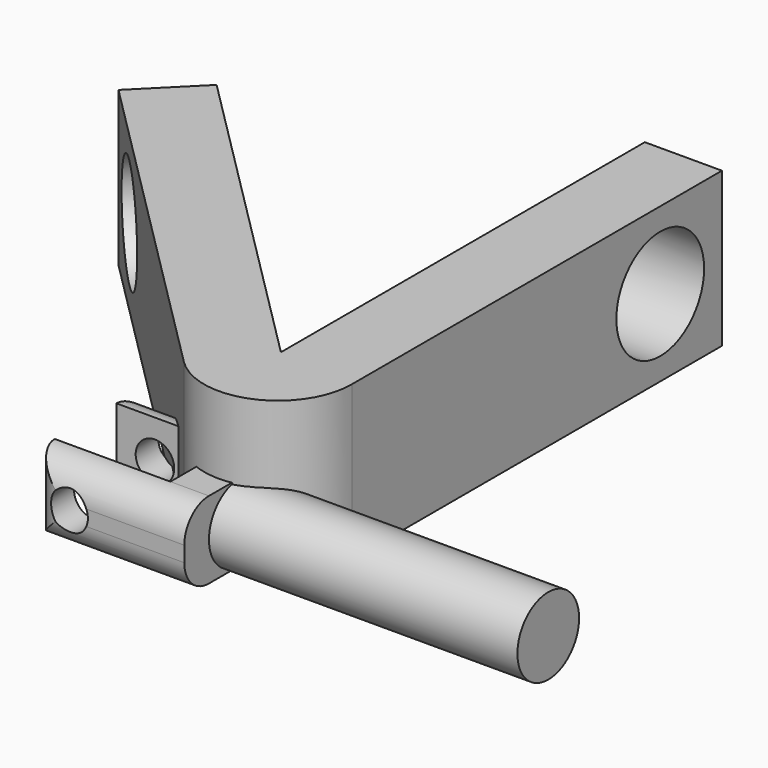
from build123d import *

# Parameters (mm, degrees)
F1_DEPTH     = 25.4
F2_R         = 9.0354062308
F3_DEPTH     = 12.7
F4_R         = 9.0297
F5_DEPTH     = 12.7
F7_DEPTH     = 12.7
F8_R         = 3.175
F9_DEPTH     = 97.9786220541
F10_R        = 6.35
F11_DEPTH    = 50.8
F12_T1_DEPTH = 50.8
F12_T3_DEPTH = 38.1


# Not quite as in the source:
# - a fillet or chamfer that OpenCascade refuses, or shapes differently, is made with other operations: its cross-section is extruded or revolved along the edge and cut away or added


with BuildPart() as f1:
    # F0 (on Top) → F1 (new body)
    with BuildSketch(Plane.XY):
        with BuildLine():
            Line((12.7, 74.9127892945), (0, 74.9127892945))
            Line((0, 74.9127892945), (0, 0))
            Line((0, 0), (-52.9713413077, 52.9713413077))
            Line((-52.9713413077, 52.9713413077), (-61.9515974288, 43.9910851867))
            Line((-61.9515974288, 43.9910851867), (-8.0700607024, -9.8904515398))
            ThreePointArc((-8.0700607024, -9.8904515398), (5.18922052, -12.5278865574), (12.7, -1.2872107055))
            Line((12.7, -1.2872107055), (12.7, 74.9127892945))
        make_face()
    extrude(amount=F1_DEPTH)

    # F2 (on Right) → F3 (cut, through all)
    with BuildSketch(Plane.YZ):
        with Locations((62.2127892945, 12.7)):
            Circle(F2_R)
    extrude(amount=F3_DEPTH, mode=Mode.SUBTRACT)

    # F4 (on face) → F5 (cut, through all)
    with BuildSketch(Plane(origin=(-8.9802561211, -8.9802561211, 0), x_dir=(0.7071067812, -0.7071067812, 0), z_dir=(-0.7071067812, -0.7071067812, 0))):
        with Locations((-62.2127892945, 12.7)):
            Circle(F4_R)
    extrude(amount=-F5_DEPTH, mode=Mode.SUBTRACT)


with BuildPart() as f7:
    # F6 (on Top) → F7 (new body)
    with BuildSketch(Plane.XY):
        Polygon((-3.8157885445, -17.9848327596), (-22.8657885445, -17.9848327596), (-22.8657885445, -23.0648327596), (2.5342114555, -23.0648327596), (2.5342114555, -0.2048327596), (-22.8657885445, -0.2048327596), (-22.8657885445, -5.2848327596), (-3.8157885445, -5.2848327596), align=None)
    extrude(amount=F7_DEPTH)

    # F8 (on face) → F9 (cut, through all)
    with BuildSketch(Plane.XZ.offset(23.0648327596)):
        with Locations((-16.5157885445, 6.35)):
            Circle(F8_R)
    extrude(amount=-F9_DEPTH, mode=Mode.SUBTRACT)

    # F12: fillet of radius 5.08 on 6 edges, made by hand

    # F12_s2 → F12_t1 (cut)
    with BuildSketch(Plane.YZ.offset(-35.5657885445)):
        with BuildLine():
            ThreePointArc((-17.9848327596, 12.7), (-21.576935208, 11.2121024484), (-23.0648327596, 7.62))
            Line((-23.0648327596, 7.62), (-23.0648327596, 12.7))
            Line((-23.0648327596, 12.7), (-17.9848327596, 12.7))
        make_face()
        with BuildLine():
            ThreePointArc((-17.9848327596, 0), (-21.576935208, 1.4878975516), (-23.0648327596, 5.08))
            Line((-23.0648327596, 5.08), (-23.0648327596, 0))
            Line((-23.0648327596, 0), (-17.9848327596, 0))
        make_face()
        with BuildLine():
            ThreePointArc((-5.2848327596, 0), (-1.6927303112, 1.4878975516), (-0.2048327596, 5.08))
            Line((-0.2048327596, 5.08), (-0.2048327596, 0))
            Line((-0.2048327596, 0), (-5.2848327596, 0))
        make_face()
        with BuildLine():
            ThreePointArc((-5.2848327596, 12.7), (-1.6927303112, 11.2121024484), (-0.2048327596, 7.62))
            Line((-0.2048327596, 7.62), (-0.2048327596, 12.7))
            Line((-0.2048327596, 12.7), (-5.2848327596, 12.7))
        make_face()
    extrude(amount=F12_T1_DEPTH, mode=Mode.SUBTRACT)

    # F12_s4 → F12_t3 (cut)
    with BuildSketch(Plane.XY.offset(-12.7)):
        with BuildLine():
            ThreePointArc((-22.8657885445, -17.9848327596), (-21.3778909929, -21.576935208), (-17.7857885445, -23.0648327596))
            Line((-17.7857885445, -23.0648327596), (-22.8657885445, -23.0648327596))
            Line((-22.8657885445, -23.0648327596), (-22.8657885445, -17.9848327596))
        make_face()
        with BuildLine():
            ThreePointArc((-22.8657885445, -5.2848327596), (-21.3778909929, -1.6927303112), (-17.7857885445, -0.2048327596))
            Line((-17.7857885445, -0.2048327596), (-22.8657885445, -0.2048327596))
            Line((-22.8657885445, -0.2048327596), (-22.8657885445, -5.2848327596))
        make_face()
    extrude(amount=F12_T3_DEPTH, mode=Mode.SUBTRACT)


with BuildPart() as f11:
    # F10 (on face) → F11 (new body)
    with BuildSketch(Plane.YZ.offset(2.5342114555)):
        with Locations((-11.6348327596, 6.35)):
            Circle(F10_R)
    extrude(amount=F11_DEPTH)


solid = Compound([f1.part, f7.part, f11.part])
